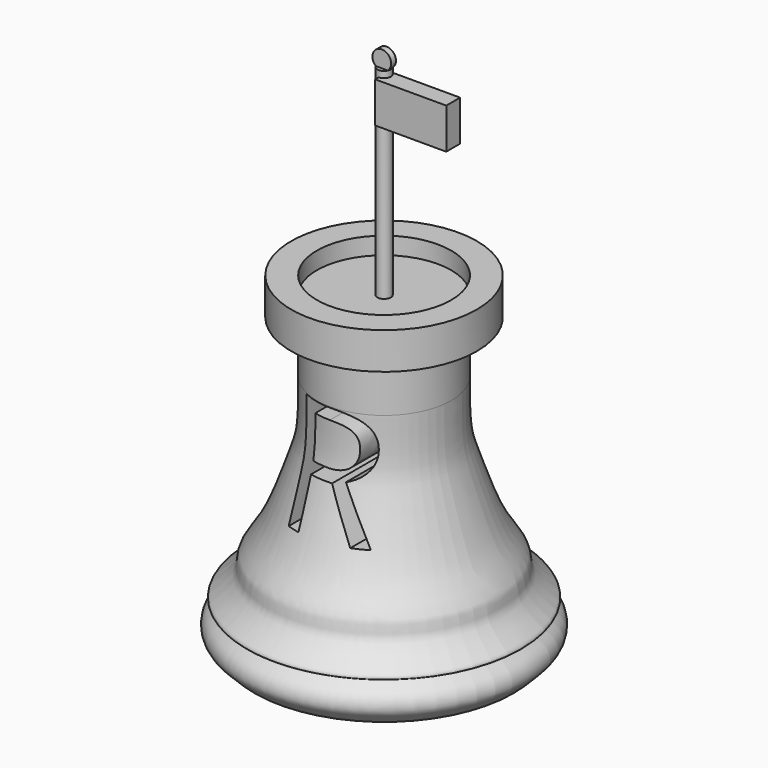
from build123d import *

# Parameters (mm, degrees)
F2_TEXT_SIZE  = 24.3055563058
F3_DEPTH      = 49
F4_R          = 1.1
F5_DEPTH      = 44
F6_W          = 11.5054104744
F6_H          = 6.570648402
F7_DEPTH      = 1.8
F7_DEPTH_BACK = 1
F8_R          = 1.5175913152
F9_DEPTH      = 0.46
F9_DEPTH_BACK = 0.51


# Not quite as in the source:
# - Text() gives the source's letters only with a copy of the font that has no kerning and outlines rounded to 1/6400 em; it was checked with that copy


with BuildPart() as f1:
    # F0 (on Front) → F1 (revolve)
    with BuildSketch(Plane.XZ):
        with BuildLine():
            Line((10.8610382304, 11.5243904293), (0, 11.5243904293))
            Line((0, 11.5243904293), (0, -38.4146347642))
            Line((0, -38.4146347642), (20.9534391761, -38.4146347642))
            add(Edge.make_bspline(
                [(20.9534391761, -38.4146347642), (21.3392316633, -38.050634438), (22.1201609191, -37.3138173322), (23.3906691736, -35.9882388647), (22.9118526166, -33.5396775878), (20.5034638475, -32.4130242588), (21.448328492, -32.0241338949), (22.6928818795, -31.6859667899), (21.4317224254, -30.4531004365), (20.3805567915, -29.7662688849), (18.4762930077, -27.6333002957), (18.8437602667, -25.3350480387), (15.4564311056, -21.6817009989), (12.3271835193, -12.0504081689), (10.8774326688, -8.0413219636), (10.8587522663, -2.0236578515), (10.8604208913, -0.5465015913), (10.8610382304, 0)],
                knots=[0, 0, 0, 0, 0.0531270374, 0.1075408649, 0.170732497, 0.2302351534, 0.2620646452, 0.3029239312, 0.3492522485, 0.4000957918, 0.4675280552, 0.5268066393, 0.6178106982, 0.7505520151, 0.841602456, 0.9413978655, 1, 1, 1, 1], degree=3))
            Line((10.8610382304, 0), (10.8610382304, 8.3813751116))
            Line((10.8610382304, 8.3813751116), (15.0166284293, 8.3813751116))
            Line((15.0166284293, 8.3813751116), (15.0166284293, 14.3181830645))
            Line((15.0166284293, 14.3181830645), (10.8610382304, 14.3181830645))
            Line((10.8610382304, 14.3181830645), (10.8610382304, 11.5243904293))
        make_face()
    revolve(axis=Axis((0, 0, 1.7461199313), (0, 0, -1)))

    # F2 (on Front) → F3 (cut)
    with BuildSketch(Plane.XZ):
        with Locations((-7.1024243007, -17.5000005402)):
            Text('R', F2_TEXT_SIZE, font='Open Sans', text_align=(TextAlign.LEFT, TextAlign.BOTTOM))
    extrude(amount=F3_DEPTH, mode=Mode.SUBTRACT)

    # F4 (on Top) → F5 (join)
    with BuildSketch(Plane.XY):
        Circle(F4_R)
    extrude(amount=F5_DEPTH)

    # F6 (on Front) → F7 (join, two sides)
    with BuildSketch(Plane.XZ) as f7_sk:
        with Locations((5.7527052372, 39.6873969585)):
            Rectangle(F6_W, F6_H)
    extrude(amount=F7_DEPTH)
    extrude(f7_sk.sketch, amount=-F7_DEPTH_BACK)

    # F8 (on Front) → F9 (join, two sides)
    with BuildSketch(Plane.XZ) as f9_sk:
        with Locations((0, 45.1765991747)):
            Circle(F8_R)
    extrude(amount=F9_DEPTH)
    extrude(f9_sk.sketch, amount=-F9_DEPTH_BACK)


solid = f1.part
